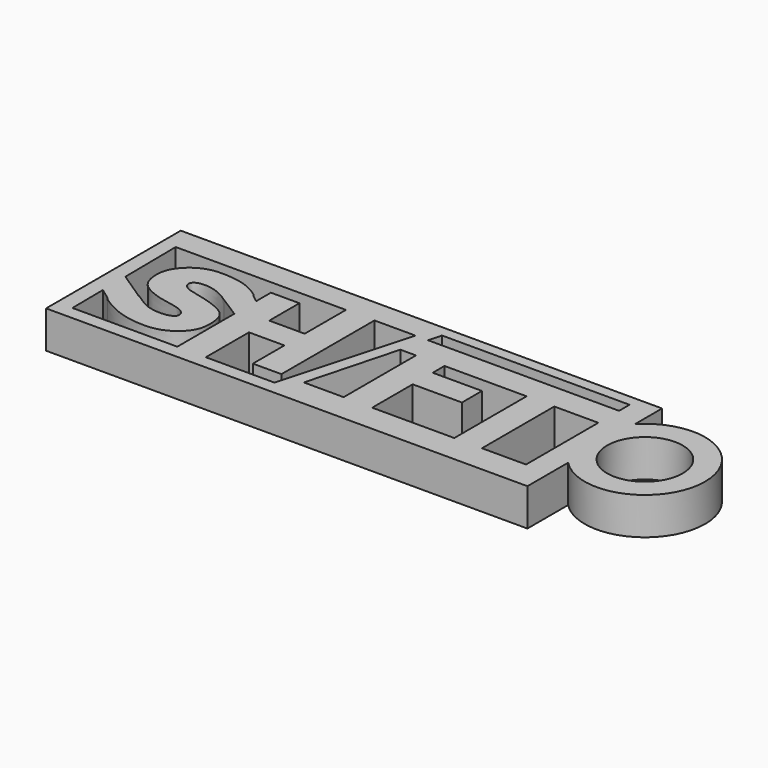
from build123d import *

# Parameters (mm, degrees)
F0_R     = 6.4346653904
F1_DEPTH = 6.35


with BuildPart() as f1:
    # F0 (on Top) → F1 (new body)
    with BuildSketch(Plane.XY):
        with BuildLine():
            Line((42.4421280622, 12.8763979301), (39.4888482988, 12.8763979301))
            Line((39.4888482988, 12.8763979301), (-39.4888482988, 12.8763979301))
            Line((-39.4888482988, 12.8763979301), (-39.4888482988, -12.8763979301))
            Line((-39.4888482988, -12.8763979301), (-39.4888482988, -15.7759096473))
            Line((-39.4888482988, -15.7759096473), (42.4421280622, -15.7759096473))
            Line((42.4421280622, -15.7759096473), (42.4421280622, -7.1135064169))
            ThreePointArc((42.4421280622, -7.1135064169), (60.0677187775, 0), (42.4421280622, 7.1135064169))
            Line((42.4421280622, 7.1135064169), (42.4421280622, 12.8763979301))
        make_face()
        with BuildLine():
            Line((-36.9513516024, -2.0756540524), (-37.0719090537, 8.7742841496))
            Line((-37.0719090537, 8.7742841496), (-8.0906844199, 8.7742841496))
            Line((-8.0906844199, 8.7742841496), (-8.0906844199, 6.4205448143))
            Line((-8.0906844199, 6.4205448143), (-8.0906844199, 0))
            Line((-8.0906844199, 0), (-14.1232470879, 0))
            Line((-14.1232470879, 0), (-14.1232470879, 6.4205448143))
            Line((-14.1232470879, 6.4205448143), (-18.9787298441, 6.4205448143))
            Line((-18.9787298441, 6.4205448143), (-18.9787298441, 3.272225149))
            Line((-18.9787298441, 3.272225149), (-20.2155560255, 4.2724418454))
            add(Edge.make_bspline(
                [(-22.5384198129, 0.9058159776), (-22.5087632242, 0.9012403563), (-22.4564231627, 1.003636113), (-20.2998909345, 4.1680794182), (-20.2137324503, 4.2468094283), (-20.2155560255, 4.2724418454)],
                knots=[0.9408554446, 0.9408554446, 0.9408554446, 0.9408554446, 0.9475987771, 0.9851160131, 0.9922654541, 0.9922654541, 0.9922654541, 0.9922654541], degree=3))
            Line((-22.5384198129, 0.9058159776), (-18.9787298441, -1.3575867051))
            Line((-18.9787298441, -1.3575867051), (-18.9787298441, -11.0218683258))
            Line((-18.9787298441, -11.0218683258), (-18.9787298441, -13.4963878203))
            Line((-18.9787298441, -13.4963878203), (-36.8244518423, -13.4963878203))
            Line((-36.8244518423, -13.4963878203), (-36.8974223987, -6.9291784173))
            Line((-36.8974223987, -6.9291784173), (-34.963618964, -8.3375107497))
            add(Edge.make_bspline(
                [(-32.2309853918, -5.2103603082), (-32.2342536022, -5.2109736525), (-32.5026233072, -5.2870456733), (-34.8780387985, -8.3306569491), (-34.9598781788, -8.3231927663), (-34.963618964, -8.3375107497)],
                knots=[0.4355467782, 0.4355467782, 0.4355467782, 0.4355467782, 0.4360630295, 0.4746738617, 0.4803443093, 0.4803443093, 0.4803443093, 0.4803443093], degree=3))
            Line((-32.2309853918, -5.2103603082), (-36.9513516024, -2.0756540524))
        make_face(mode=Mode.SUBTRACT)
        Polygon((-3.2352029779, 8.7742841496), (3.757656788, 8.7742841496), (-2.4286360377, -13.4963878203), (-14.1232470879, -13.4963878203), (-14.1232470879, -11.0218693809), (-14.1232470879, -4.3203692259), (-8.0906844199, -4.3203692259), (-8.0906844199, -11.0218693809), (-3.2352029779, -11.0218693809), (-3.2352029779, 6.4205437592), align=None, mode=Mode.SUBTRACT)
        Polygon((7.3585736133, -11.0218693809), (0.585847945, -11.0218693809), (4.7024635713, 4.360642626), (7.3585736133, 4.360642626), (7.3585736133, -8.7344424174), align=None, mode=Mode.SUBTRACT)
        Polygon((26.1919542714, 4.360642626), (26.1919542714, -8.7344424174), (26.1919542714, -11.0218693809), (12.214054124, -11.0218693809), (12.214054124, -8.7344424174), (12.214054124, -2.4076042538), (20.6007964476, -2.4076042538), (20.6007964476, 1.8593341737), (12.214054124, 1.8593341737), (12.214054124, 4.360642626), align=None, mode=Mode.SUBTRACT)
        Polygon((38.4009263977, 4.360642626), (38.4009263977, -11.0218693809), (30.9003021135, -11.0218693809), (30.9003021135, -8.7344424174), (30.9003021135, 4.360642626), (36.1971899434, 4.360642626), align=None, mode=Mode.SUBTRACT)
        with Locations((49.8194545507, 0)):
            Circle(F0_R, mode=Mode.SUBTRACT)
        Polygon((5.8836273277, 8.7742841496), (6.4796276889, 11.001352097), (38.4009263977, 11.001352097), (38.4009263977, 8.7742841496), (36.1971899434, 8.7742841496), (7.3585736133, 8.7742841496), align=None, mode=Mode.SUBTRACT)
        with BuildLine():
            Line((-32.1797840297, -5.244362168), (-32.2309853918, -5.2103603082))
            add(Edge.make_bspline(
                [(-32.2309853918, -5.2103603082), (-32.2342536022, -5.2109736525), (-32.5026233072, -5.2870456733), (-34.8780387985, -8.3306569491), (-34.9598781788, -8.3231927663), (-34.963618964, -8.3375107497)],
                knots=[0.4355467782, 0.4355467782, 0.4355467782, 0.4355467782, 0.4360630295, 0.4746738617, 0.4803443093, 0.4803443093, 0.4803443093, 0.4803443093], degree=3))
            add(Edge.make_bspline(
                [(-34.963618964, -8.3375107497), (-34.9675743656, -8.3526501853), (-34.94912, -8.5187549568), (-33.3696351013, -9.6007944416), (-30.7920969463, -10.8958063848), (-26.8035065017, -11.6393224595), (-22.862499267, -11.1518414802), (-19.5984169566, -8.1691908864), (-19.6017291407, -4.5553773395), (-20.4674273936, -1.5312135148), (-26.7401677603, 0.0475188317), (-28.2464831836, 0.2865770189), (-29.3057058095, 1.2745574964), (-28.9466933204, 2.4241158437), (-27.2521069685, 2.7924557318), (-24.9448859469, 2.3970789833), (-23.0875367983, 1.3142896199), (-22.7543139439, 1.0055321165), (-22.5757111205, 0.9115695355), (-22.5384198129, 0.9058159776)],
                knots=[0.4803443093, 0.4803443093, 0.4803443093, 0.4803443093, 0.4863400822, 0.5112582455, 0.5449682746, 0.5833039505, 0.6212246257, 0.6596699414, 0.6947214559, 0.727122413, 0.774281972, 0.7988549754, 0.8196537682, 0.8379758627, 0.8618457815, 0.8920874529, 0.9196965763, 0.9323761252, 0.9408554446, 0.9408554446, 0.9408554446, 0.9408554446], degree=3))
            add(Edge.make_bspline(
                [(-22.5384198129, 0.9058159776), (-22.5087632242, 0.9012403563), (-22.4564231627, 1.003636113), (-20.2998909345, 4.1680794182), (-20.2137324503, 4.2468094283), (-20.2155560255, 4.2724418454)],
                knots=[0.9408554446, 0.9408554446, 0.9408554446, 0.9408554446, 0.9475987771, 0.9851160131, 0.9922654541, 0.9922654541, 0.9922654541, 0.9922654541], degree=3))
            add(Edge.make_bspline(
                [(-20.2155560255, 4.2724418454), (-20.2175288408, 4.3001720003), (-20.2377762384, 4.3431530092), (-20.3018076718, 4.4104824774)],
                knots=[0.9922654541, 0.9922654541, 0.9922654541, 0.9922654541, 1, 1, 1, 1], degree=3))
            add(Edge.make_bspline(
                [(-20.3018076718, 4.4104824774), (-20.5611843452, 4.6832187345), (-22.7532194208, 6.1902747016), (-26.5857065373, 6.8273013596), (-30.5682744913, 6.6366330017), (-34.0772532991, 3.5349548203), (-34.2377624912, -0.0216028843), (-33.2232441235, -2.6818995712), (-29.0735436506, -4.2584680685), (-25.9931449346, -4.5345033939), (-24.4088698097, -5.5757988745), (-24.4735796107, -6.9657080374), (-26.77069563, -7.515523238), (-29.8441369576, -6.9840985647), (-31.926415002, -5.2512697169), (-32.1542497767, -5.2697193823), (-32.1797840297, -5.244362168)],
                knots=[0, 0, 0, 0, 0.0313308742, 0.0702363738, 0.108023624, 0.1476505721, 0.1824883473, 0.2133365645, 0.2527583853, 0.2871936467, 0.3116497664, 0.3304953042, 0.3577411479, 0.3930772692, 0.4232438974, 0.4310210993, 0.4310210993, 0.4310210993, 0.4310210993], degree=3))
        make_face()
    extrude(amount=F1_DEPTH)


solid = f1.part
